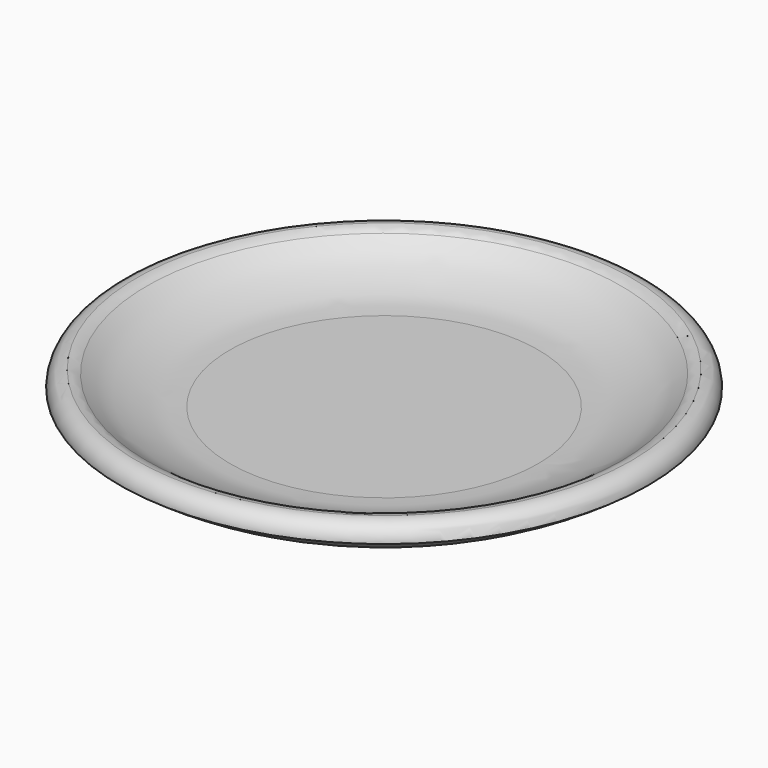
from build123d import *

# Parameters (mm, degrees)
F0_R     = 25.4
F0_R_2   = 22.225
F1_DEPTH = 6.35
F2_DEPTH = 3.175
F3_R     = 1.5875
F4_R     = 1.58749
F5_R     = 12.7


# Not quite as in the source:
# - a fillet or chamfer that OpenCascade refuses, or shapes differently, is made with other operations: its cross-section is extruded or revolved along the edge and cut away or added
# - a fillet or chamfer is up to 0.001 mm smaller than in the source, because OpenCascade refuses the exact size


with BuildPart() as f1:
    # F0 (on Top) → F1 (new body)
    with BuildSketch(Plane.XY):
        Circle(F0_R)
        Circle(F0_R_2, mode=Mode.SUBTRACT)
    extrude(amount=F1_DEPTH)

    # F0 (on Top) → F2 (join)
    with BuildSketch(Plane.XY):
        Circle(F0_R_2)
    extrude(amount=F2_DEPTH)

    # F3
    f3_edges = [f1.edges().sort_by_distance(p)[0] for p in [
        (-22.225, 0, 6.35),
    ]]
    fillet(f3_edges, radius=F3_R)

    # F4 (radius 1.5875 in the source; OpenCascade refuses exactly that, so slightly less here)
    f4_edges = [f1.edges().sort_by_distance(p)[0] for p in [
        (-25.4, 0, 6.35),
    ]]
    fillet(f4_edges, radius=F4_R)

    # F5
    f5_edges = [f1.edges().sort_by_distance(p)[0] for p in [
        (-22.225, 0, 3.175),
    ]]
    fillet(f5_edges, radius=F5_R)

    # F6: fillet of radius 25.4 on 1 edges, made by hand

    # F6_s1 → F6_t2 (revolve, cut)
    with BuildSketch(Plane.XZ):
        with BuildLine():
            ThreePointArc((25.4, 4.76251), (18.3699099141, 1.219923015), (10.5927718158, 0))
            Line((10.5927718158, 0), (10.5927718158, -0.508))
            Line((10.5927718158, -0.508), (25.4, -0.508))
            Line((25.4, -0.508), (25.908, 0))
            ThreePointArc((25.908, 0), (25.908, 2.381255), (25.6961445637, 4.3497602))
            Line((25.6961445637, 4.3497602), (25.4, 4.76251))
        make_face()
    revolve(axis=Axis((0, 0, 0), (0, 0, 1)), mode=Mode.SUBTRACT)


solid = f1.part
